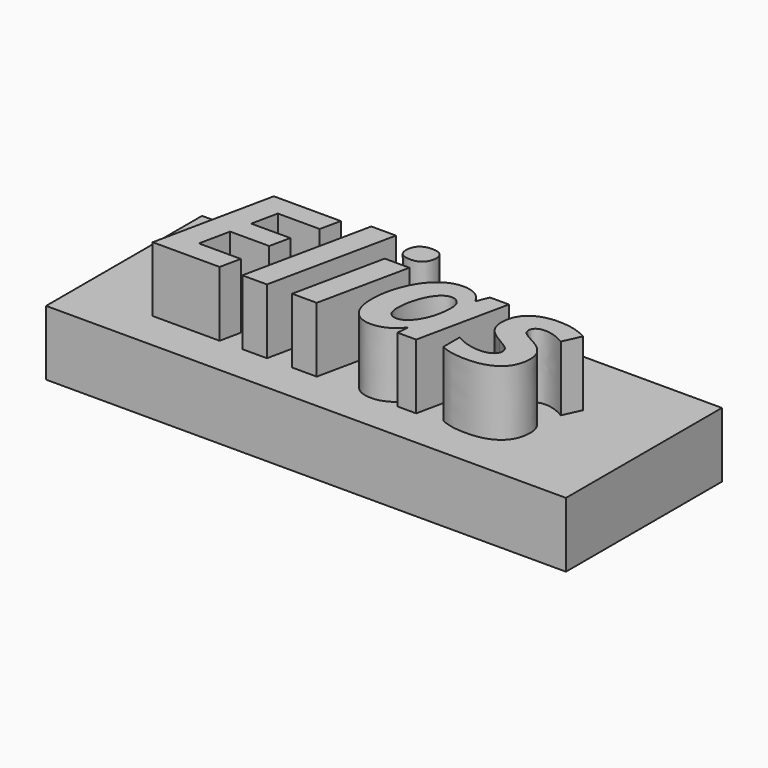
from build123d import *

# Parameters (mm, degrees)
F0_W         = 101.6
F0_H         = 38.1
F1_DEPTH     = 12.7
F2_TEXT_SIZE = 32.7778773175
F3_DEPTH     = 12.7


# Not quite as in the source:
# - Text() gives the source's letters only with a copy of the font that has no kerning and outlines rounded to 1/6400 em; it was checked with that copy


with BuildPart() as f1:
    # F0 (on Top) → F1 (new body)
    with BuildSketch(Plane.XY):
        Rectangle(F0_W, F0_H)
    extrude(amount=F1_DEPTH)

    # F2 (on face) → F3 (join)
    with BuildSketch(Plane.XY.offset(12.7)):
        with Locations((-36.8391312659, -11.5122301504)):
            Text('Elias', F2_TEXT_SIZE, font='Open Sans', font_style=FontStyle.BOLDITALIC, text_align=(TextAlign.LEFT, TextAlign.BOTTOM))
    extrude(amount=F3_DEPTH)


solid = f1.part
